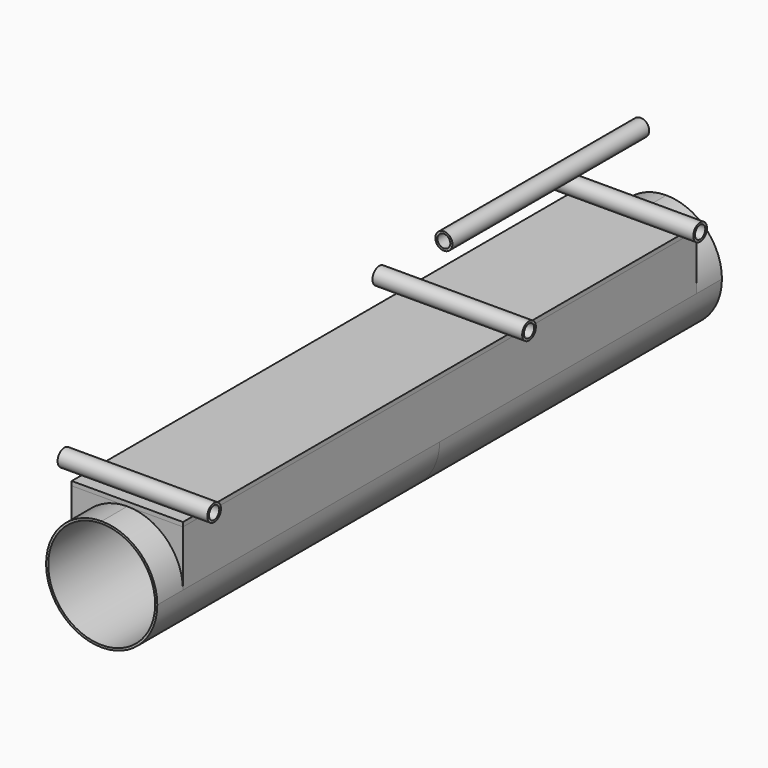
from build123d import *

# Parameters (mm, degrees)
F1_DEPTH = 165
F2_DEPTH = 150
F3_DEPTH = 150
F5_START = -35
F4_R     = 4
F4_R_2   = 3
F5_DEPTH = 115
F6_R     = 4
F6_R_2   = 3
F7_DEPTH = 35


with BuildPart() as f1:
    # F0 (on Front) → F1 (new body, symmetric)
    with BuildSketch(Plane.XZ):
        with BuildLine():
            ThreePointArc((0, 26), (-18.3847763109, 18.3847763109), (-26, 0))
            Line((-26, 0), (-25, 0))
            ThreePointArc((-25, 0), (0, 25), (25, 0))
            Line((25, 0), (26, 0))
            ThreePointArc((26, 0), (18.3847763109, 18.3847763109), (0, 26))
        make_face()
        with BuildLine():
            Line((-25, 0), (-26, 0))
            ThreePointArc((-26, 0), (0, -26), (26, 0))
            Line((26, 0), (25, 0))
            ThreePointArc((25, 0), (0, -25), (-25, 0))
        make_face()
    extrude(amount=F1_DEPTH, both=True)


with BuildPart() as f2:
    # F0 (on Front) → F2 (new body, symmetric)
    with BuildSketch(Plane.XZ):
        Polygon((-26, 26), (0, 26), (26, 26), (26, 28), (-26, 28), align=None)
    extrude(amount=F2_DEPTH, both=True)


with BuildPart() as f3:
    # F0 (on Front) → F3 (new body, symmetric)
    with BuildSketch(Plane.XZ):
        with BuildLine():
            ThreePointArc((0, 26), (18.3847763109, 18.3847763109), (26, 0))
            Line((26, 0), (26, 26))
            Line((26, 26), (0, 26))
        make_face()
    extrude(amount=F3_DEPTH, both=True)


with BuildPart() as f3b:
    # F0 (on Front) → F3, piece 2 (new body, symmetric)
    with BuildSketch(Plane.XZ):
        with BuildLine():
            Line((-26, 26), (-26, 0))
            ThreePointArc((-26, 0), (-18.3847763109, 18.3847763109), (0, 26))
            Line((0, 26), (-26, 26))
        make_face()
    extrude(amount=F3_DEPTH, both=True)


with BuildPart() as f5:
    # F4 (on Front) → F5 (new body)
    with BuildSketch(Plane.XZ.offset(F5_START)):
        with Locations((0, 60)):
            Circle(F4_R)
        with Locations((0, 60)):
            Circle(F4_R_2, mode=Mode.SUBTRACT)
    extrude(amount=-F5_DEPTH)


with BuildPart() as f7:
    # F6 (on Right) → F7 (new body, symmetric)
    with BuildSketch(Plane.YZ):
        with Locations((-143.0319845676, 32)):
            Circle(F6_R)
        with Locations((-143.0319845676, 32)):
            Circle(F6_R_2, mode=Mode.SUBTRACT)
    extrude(amount=F7_DEPTH, both=True)


with BuildPart() as f7b:
    # F6 (on Right) → F7, piece 2 (new body, symmetric)
    with BuildSketch(Plane.YZ):
        with Locations((141.0174369812, 32)):
            Circle(F6_R)
        with Locations((141.0174369812, 32)):
            Circle(F6_R_2, mode=Mode.SUBTRACT)
    extrude(amount=F7_DEPTH, both=True)


with BuildPart() as f7c:
    # F6 (on Right) → F7, piece 3 (new body, symmetric)
    with BuildSketch(Plane.YZ):
        with Locations((41.0174369812, 32)):
            Circle(F6_R)
        with Locations((41.0174369812, 32)):
            Circle(F6_R_2, mode=Mode.SUBTRACT)
    extrude(amount=F7_DEPTH, both=True)


solid = Compound([f1.part, f2.part, f3.part, f3b.part, f5.part, f7.part, f7b.part, f7c.part])
